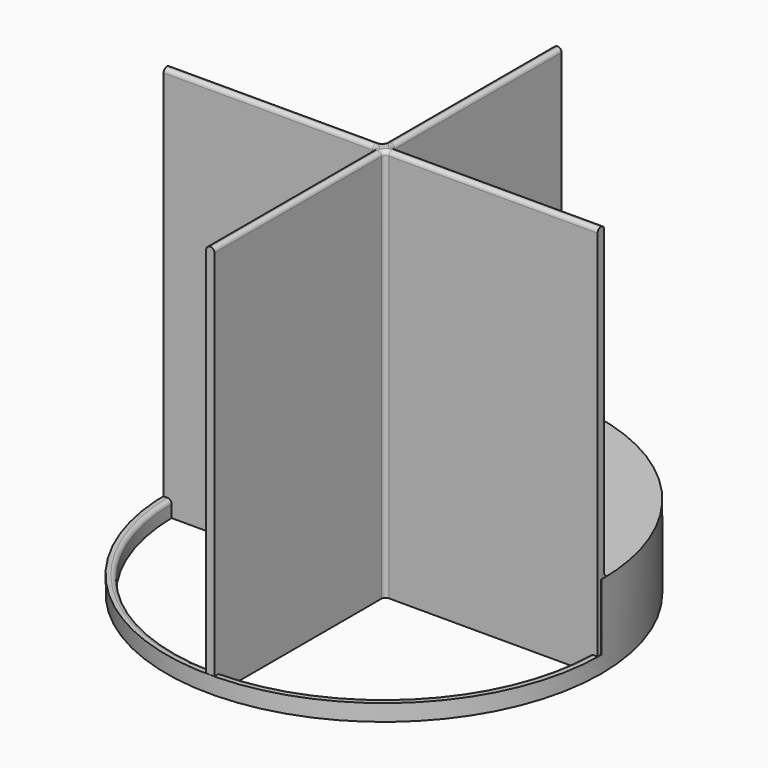
from build123d import *

# Parameters (mm, degrees)
F0_R     = 52.5
F0_R_2   = 50.5
F1_DEPTH = 4
F2_W     = 2
F2_H     = 51.4
F2_W_2   = 51.4
F2_H_2   = 2
F3_DEPTH = 95
F5_DEPTH = 20
F6_F1_R  = 1
F6_F2_R  = 1
F6_F3_R  = 0.9999
F7_R     = 0.99999


# Not quite as in the source:
# - a fillet or chamfer is up to 0.001 mm smaller than in the source, because OpenCascade refuses the exact size


with BuildPart() as f1:
    # F0 (on Top) → F1 (new body)
    with BuildSketch(Plane.XY):
        Circle(F0_R)
        Circle(F0_R_2, mode=Mode.SUBTRACT)
    extrude(amount=F1_DEPTH)

    # F2 (on Top) → F3 (join)
    with BuildSketch(Plane.XY):
        with Locations((0, -26.7)):
            Rectangle(F2_W, F2_H)
        with Locations((-26.7, 0)):
            Rectangle(F2_W_2, F2_H_2)
        Rectangle(F2_W, F2_H_2)
        with Locations((26.7, 0)):
            Rectangle(F2_W_2, F2_H_2)
        with Locations((0, 26.7)):
            Rectangle(F2_W, F2_H)
    extrude(amount=F3_DEPTH)

    # F4 (on Top) → F5 (join)
    with BuildSketch(Plane.XY):
        with BuildLine():
            Line((0, 0), (52.5, 0))
            ThreePointArc((52.5, 0), (37.1231060123, 37.1231060123), (0, 52.5))
            Line((0, 52.5), (0, 0))
        make_face()
    extrude(amount=F5_DEPTH)

    # F6: fillet of radius 1 on 13 edges, made by hand

    # F6_f1
    f6_f1_edges = [f1.edges().sort_by_distance(p)[0] for p in [
        (1, 1, 57.5),
        (26.7, 1, 20),
        (1, 26.7, 20),
        (-1, 1, 47.5),
        (1, -1, 47.5),
        (-1, -1, 47.5),
    ]]
    fillet(f6_f1_edges, radius=F6_F1_R)

    # F6_f2
    f6_f2_edges = [f1.edges().sort_by_distance(p)[0] for p in [
        (-27.2, 1, 95),
        (-35.7088924499, -35.7088924499, 4),
        (35.7088924499, -35.7088924499, 4),
        (-35.7088924499, 35.7088924499, 0),
        (-35.7088924499, 35.7088924499, 4),
        (-1.2928932188, 1.2928932188, 95),
    ]]
    fillet(f6_f2_edges, radius=F6_F2_R)

    # F6_f3 (radius 1 in the source; OpenCascade refuses exactly that, so slightly less here)
    f6_f3_edges = [f1.edges().sort_by_distance(p)[0] for p in [
        (1, 27.2, 95),
        (27.2, 1, 95),
        (1.2928932188, 1.2928932188, 95),
    ]]
    fillet(f6_f3_edges, radius=F6_F3_R)

    # F7 (radius 1 in the source; OpenCascade refuses exactly that, so slightly less here)
    f7_edges = [f1.edges().sort_by_distance(p)[0] for p in [
        (1, -27.2, 95),
        (-1, -27.2, 95),
        (-27.2, -1, 95),
        (27.2, -1, 95),
        (1.292893, -1.292893, 95),
        (-1.292893, -1.292893, 95),
    ]]
    fillet(f7_edges, radius=F7_R)


solid = f1.part
